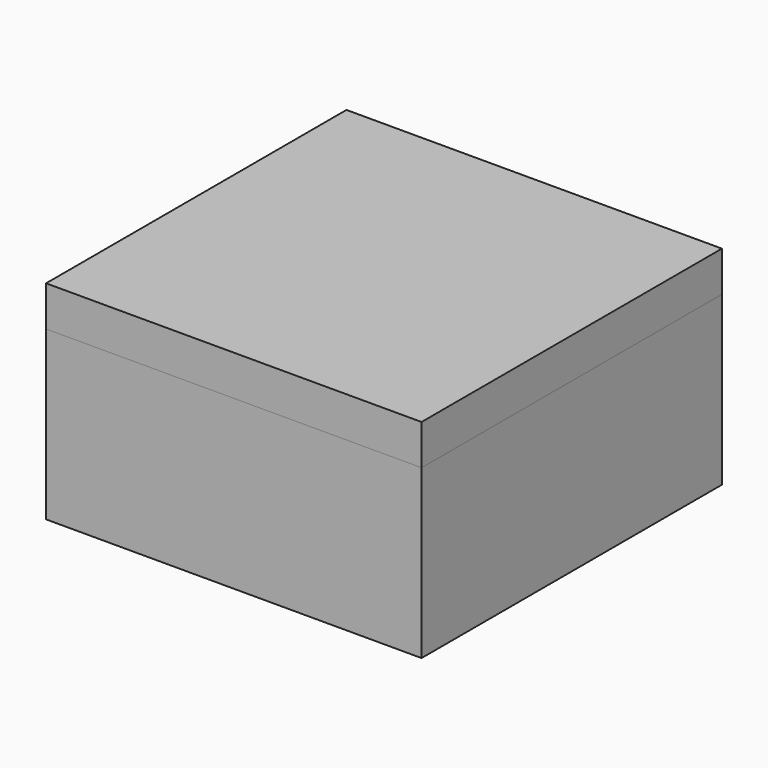
from build123d import *

# Parameters (mm, degrees)
F0_W     = 22.225
F0_H     = 9.921875
F1_DEPTH = 22.225
F2_W     = 22.225
F2_H     = 2.38125
F3_DEPTH = 22.225


# Not quite as in the source:
# - a length typed as a fraction of an inch, garbled in the dataset ("3 / 203.2 mm" for 3/8 in), is restored
# - a feature names something its author has since deleted; it is built from what else it names


with BuildPart() as f1:
    # F0 (on Front) → F1 (new body)
    with BuildSketch(Plane.XZ):
        with Locations((11.1125, 4.9609375)):
            Rectangle(F0_W, F0_H)
    extrude(amount=F1_DEPTH)


with BuildPart() as f3:
    # F2 (on Front) → F3 (new body)
    with BuildSketch(Plane.XZ):
        with Locations((11.1125, 11.1125)):
            Rectangle(F2_W, F2_H)
    extrude(amount=F3_DEPTH)


solid = Compound([f1.part, f3.part])
